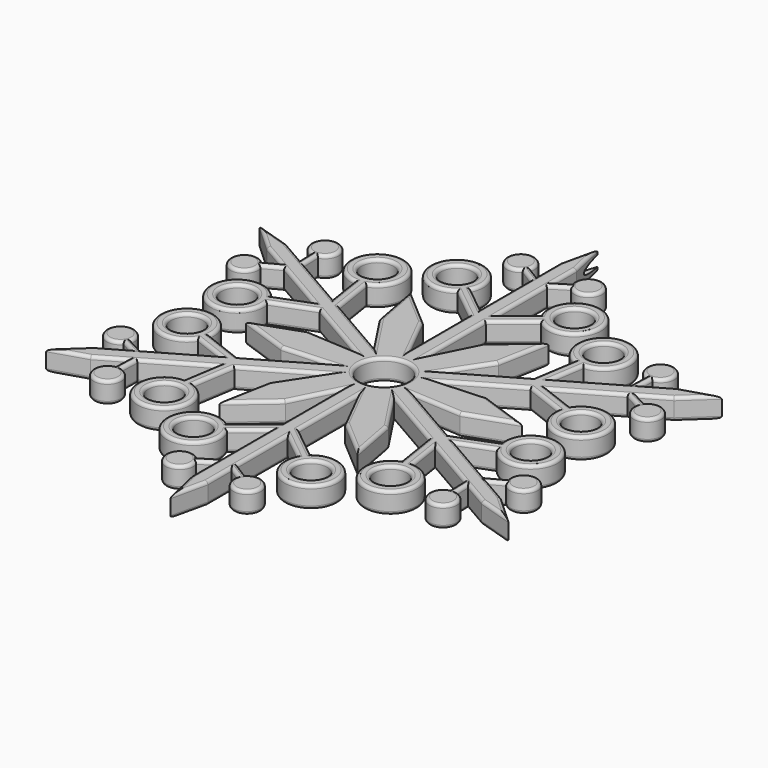
from build123d import *

# Parameters (mm, degrees)
F0_R     = 1.5
F1_DEPTH = 1
F3_COUNT = 6
F4_R     = 2.25
F5_DEPTH = 2.001
F6_R     = 0.29999
F8_R     = 0.5
F9_DEPTH = 3


# Not quite as in the source:
# - a fillet or chamfer is up to 0.001 mm smaller than in the source, because OpenCascade refuses the exact size


with BuildPart() as f1:
    # F0 (on Top) → F1 (new body, symmetric)
    with BuildSketch(Plane.XY):
        with BuildLine():
            Line((0.7675196002, 21.582075705), (0, 25))
            Line((0, 25), (-0.7675196002, 21.582075705))
            Line((-0.7675196002, 21.582075705), (-0.7675196002, 18.8360231686))
            Line((-0.7675196002, 18.8360231686), (-1.9404436058, 19.5647595556))
            ThreePointArc((-1.9404436058, 19.5647595556), (-4.2601998947, 20.6528344986), (-2.2570854353, 19.0551146284))
            Line((-2.2570854353, 19.0551146284), (-0.7675196002, 18.1296490231))
            Line((-0.7675196002, 18.1296490231), (-0.7675196002, 12.2385434307))
            Line((-0.7675196002, 12.2385434307), (-3.2830186101, 14.2674330896))
            ThreePointArc((-3.2830186101, 14.2674330896), (-7.4494710439, 16.9855432476), (-3.9108200753, 13.4890595802))
            Line((-3.9108200753, 13.4890595802), (-0.7675196002, 10.9538131723))
            Line((-0.7675196002, 10.9538131723), (-0.7675196002, 4.0098051105))
            Line((-0.7675196002, 4.0098051105), (-2.8030935325, 8.0551004166))
            Line((-2.8030935325, 8.0551004166), (-6.46553243, 11.1986306667))
            Line((-6.46553243, 11.1986306667), (0, 0))
            Line((0, 0), (6.46553243, 11.1986306667))
            Line((6.46553243, 11.1986306667), (2.8030935325, 8.0551004166))
            Line((2.8030935325, 8.0551004166), (0.7675196002, 4.0098051105))
            Line((0.7675196002, 4.0098051105), (0.7675196002, 10.9538131723))
            Line((0.7675196002, 10.9538131723), (3.9108200753, 13.4890595802))
            ThreePointArc((3.9108200753, 13.4890595802), (7.4494710439, 16.9855432476), (3.2830186101, 14.2674330896))
            Line((3.2830186101, 14.2674330896), (0.7675196002, 12.2385434307))
            Line((0.7675196002, 12.2385434307), (0.7675196002, 18.1296490231))
            Line((0.7675196002, 18.1296490231), (2.2570854353, 19.0551146284))
            ThreePointArc((2.2570854353, 19.0551146284), (4.2601998947, 20.6528344986), (1.9404436058, 19.5647595556))
            Line((1.9404436058, 19.5647595556), (0.7675196002, 18.8360231686))
            Line((0.7675196002, 18.8360231686), (0.7675196002, 21.582075705))
        make_face()
        with Locations((-5.5035372702, 15.4160395845)):
            Circle(F0_R, mode=Mode.SUBTRACT)
        with Locations((5.5035372702, 15.4160395845)):
            Circle(F0_R, mode=Mode.SUBTRACT)
    extrude(amount=F1_DEPTH, both=True)

    # F3: F1 ×6 about axis
    f3_axis = Axis((0, 0, 6.4609721303), (0, 0, 1))


with BuildPart() as f1_1:
    add(f1.part)
    for i in range(1, F3_COUNT):
        add(f1.part.rotate(f3_axis, i * 360 / F3_COUNT))

    # F4 (on face) → F5 (cut, through all)
    with BuildSketch(Plane.XY.offset(1)):
        Circle(F4_R)
    extrude(amount=-F5_DEPTH, mode=Mode.SUBTRACT)

    # F6 (radius 0.3 in the source; OpenCascade refuses exactly that, so slightly less here)
    f6_edges = [f1_1.edges().sort_by_distance(p)[0] for p in [
        (4.2602, 20.652834, 1),
        (1.512303, 18.592382, 1),
        (1.353982, 19.200391, 1),
        (0.76752, 15.184096, 1),
        (0.76752, 20.209049, 1),
        (2.025269, 13.252988, 1),
        (0.38376, 23.291038, 1),
        (7.449471, 16.985543, 1),
        (-0.38376, 23.291038, 1),
        (2.33917, 12.221436, 1),
        (-0.76752, 20.209049, 1),
        (0.76752, 7.481809, 1),
        (-1.353982, 19.200391, 1),
        (1.785307, 6.032453, 1),
        (-4.2602, 20.652834, 1),
        (4.634313, 9.626866, 1),
        (-1.512303, 18.592382, 1),
        (6.019954, 8.826866, 1),
        (-0.76752, 15.184096, 1),
        (4.331604, 4.562347, 1),
        (-2.025269, 13.252988, 1),
        (6.095677, 4.405596, 1),
        (-7.449471, 16.985543, 1),
        (9.414489, 8.136499, 1),
        (-2.33917, 12.221436, 1),
        (10.985176, 14.944203, 1),
        (-0.76752, 7.481809, 1),
        (10.46479, 8.380429, 1),
        (-1.785307, 6.032453, 1),
        (12.766053, 8.25674, 1),
        (-4.634313, 9.626866, 1),
        (15.345324, 10.605883, 1),
        (-6.019954, 8.826866, 1),
        (15.755779, 14.015859, 1),
        (-4.331604, 4.562347, 1),
        (15.951036, 10.772778, 1),
        (-6.095677, 4.405596, 1),
        (17.11779, 10.769216, 1),
        (-9.414489, 8.136499, 1),
        (19.978751, 11.977865, 1),
        (-10.985176, 14.944203, 1),
        (20.36251, 11.313173, 1),
        (-10.46479, 8.380429, 1),
        (17.88531, 9.439833, 1),
        (-12.766053, 8.25674, 1),
        (17.305017, 8.427613, 1),
        (-15.345324, 10.605883, 1),
        (20.015979, 6.636976, 1),
        (-15.755779, 14.015859, 1),
        (16.857626, 7.986499, 1),
        (-15.951036, 10.772778, 1),
        (13.533573, 6.927357, 1),
        (-17.11779, 10.769216, 1),
        (12.490059, 4.87256, 1),
        (-19.978751, 11.977865, 1),
        (18.434647, 2.04134, 1),
        (-20.36251, 11.313173, 1),
        (11.753659, 4.084938, 1),
        (-17.88531, 9.439833, 1),
        (6.863197, 3.076213, 1),
        (-17.305017, 8.427613, 1),
        (6.116911, 1.470106, 1),
        (-20.015979, 6.636976, 1),
        (10.654267, 0.8, 1),
        (-16.857626, 7.986499, 1),
        (10.654267, -0.8, 1),
        (-13.533573, 6.927357, 1),
        (6.116911, -1.470106, 1),
        (-12.490059, 4.87256, 1),
        (6.863197, -3.076213, 1),
        (-18.434647, 2.04134, 1),
        (11.753659, -4.084938, 1),
        (-11.753659, 4.084938, 1),
        (18.434647, -2.04134, 1),
        (-6.863197, 3.076213, 1),
        (12.490059, -4.87256, 1),
        (-6.116911, 1.470106, 1),
        (13.533573, -6.927357, 1),
        (-10.654267, 0.8, 1),
        (16.857626, -7.986499, 1),
        (-10.654267, -0.8, 1),
        (20.015979, -6.636976, 1),
        (-6.116911, -1.470106, 1),
        (17.305017, -8.427613, 1),
        (-6.863197, -3.076213, 1),
        (17.88531, -9.439833, 1),
        (-11.753659, -4.084938, 1),
        (20.36251, -11.313173, 1),
        (-18.434647, -2.04134, 1),
        (19.978751, -11.977865, 1),
        (-12.490059, -4.87256, 1),
        (17.11779, -10.769216, 1),
        (-13.533573, -6.927357, 1),
        (15.951036, -10.772778, 1),
        (-16.857626, -7.986499, 1),
        (15.755779, -14.015859, 1),
        (-20.015979, -6.636976, 1),
        (15.345324, -10.605883, 1),
        (-17.305017, -8.427613, 1),
        (12.766053, -8.25674, 1),
        (-17.88531, -9.439833, 1),
        (10.46479, -8.380429, 1),
        (-20.36251, -11.313173, 1),
        (10.985176, -14.944203, 1),
        (-19.978751, -11.977865, 1),
        (9.414489, -8.136499, 1),
        (-17.11779, -10.769216, 1),
        (6.095677, -4.405596, 1),
        (-15.951036, -10.772778, 1),
        (4.331604, -4.562347, 1),
        (-15.755779, -14.015859, 1),
        (6.019954, -8.826866, 1),
        (-15.345324, -10.605883, 1),
        (4.634313, -9.626866, 1),
        (-12.766053, -8.25674, 1),
        (1.785307, -6.032453, 1),
        (-10.46479, -8.380429, 1),
        (0.76752, -7.481809, 1),
        (-10.985176, -14.944203, 1),
        (2.33917, -12.221436, 1),
        (-9.414489, -8.136499, 1),
        (7.449471, -16.985543, 1),
        (-6.095677, -4.405596, 1),
        (2.025269, -13.252988, 1),
        (-4.331604, -4.562347, 1),
        (0.76752, -15.184096, 1),
        (-6.019954, -8.826866, 1),
        (1.512303, -18.592382, 1),
        (-4.634313, -9.626866, 1),
        (4.2602, -20.652834, 1),
        (-1.785307, -6.032453, 1),
        (1.353982, -19.200391, 1),
        (-0.76752, -7.481809, 1),
        (0.76752, -20.209049, 1),
        (-2.33917, -12.221436, 1),
        (0.38376, -23.291038, 1),
        (-7.449471, -16.985543, 1),
        (-0.38376, -23.291038, 1),
        (-2.025269, -13.252988, 1),
        (-0.76752, -20.209049, 1),
        (-0.76752, -15.184096, 1),
        (-1.353982, -19.200391, 1),
        (-1.512303, -18.592382, 1),
        (-4.2602, -20.652834, 1),
        (-9.848913, -13.773261, 1),
        (-4.003537, -15.41604, 1),
        (-15.352451, -4.240855, 1),
        (7.003537, -15.41604, 1),
        (11.348913, -11.175185, 1),
        (16.852451, -1.642779, 1),
        (-16.852451, 1.642779, 1),
        (-11.348913, 11.175185, 1),
        (-7.003537, 15.41604, 1),
        (-2.25, 0, 1),
        (15.352451, 4.240855, 1),
        (4.003537, 15.41604, 1),
        (9.848913, 13.773261, 1),
        (4.2602, 20.652834, -1),
        (1.512303, 18.592382, -1),
        (1.353982, 19.200391, -1),
        (0.76752, 15.184096, -1),
        (0.76752, 20.209049, -1),
        (2.025269, 13.252988, -1),
        (0.38376, 23.291038, -1),
        (7.449471, 16.985543, -1),
        (-0.38376, 23.291038, -1),
        (2.33917, 12.221436, -1),
        (-0.76752, 20.209049, -1),
        (0.76752, 7.481809, -1),
        (-1.353982, 19.200391, -1),
        (1.785307, 6.032453, -1),
        (-4.2602, 20.652834, -1),
        (4.634313, 9.626866, -1),
        (-1.512303, 18.592382, -1),
        (6.019954, 8.826866, -1),
        (-0.76752, 15.184096, -1),
        (4.331604, 4.562347, -1),
        (-2.025269, 13.252988, -1),
        (6.095677, 4.405596, -1),
        (-7.449471, 16.985543, -1),
        (9.414489, 8.136499, -1),
        (-2.33917, 12.221436, -1),
        (10.985176, 14.944203, -1),
        (-0.76752, 7.481809, -1),
        (10.46479, 8.380429, -1),
        (-1.785307, 6.032453, -1),
        (12.766053, 8.25674, -1),
        (-4.634313, 9.626866, -1),
        (15.345324, 10.605883, -1),
        (-6.019954, 8.826866, -1),
        (15.755779, 14.015859, -1),
        (-4.331604, 4.562347, -1),
        (15.951036, 10.772778, -1),
        (-6.095677, 4.405596, -1),
        (17.11779, 10.769216, -1),
        (-9.414489, 8.136499, -1),
        (19.978751, 11.977865, -1),
        (-10.985176, 14.944203, -1),
        (20.36251, 11.313173, -1),
        (-10.46479, 8.380429, -1),
        (17.88531, 9.439833, -1),
        (-12.766053, 8.25674, -1),
        (17.305017, 8.427613, -1),
        (-15.345324, 10.605883, -1),
        (20.015979, 6.636976, -1),
        (-15.755779, 14.015859, -1),
        (16.857626, 7.986499, -1),
        (-15.951036, 10.772778, -1),
        (13.533573, 6.927357, -1),
        (-17.11779, 10.769216, -1),
        (12.490059, 4.87256, -1),
        (-19.978751, 11.977865, -1),
        (18.434647, 2.04134, -1),
        (-20.36251, 11.313173, -1),
        (11.753659, 4.084938, -1),
        (-17.88531, 9.439833, -1),
        (6.863197, 3.076213, -1),
        (-17.305017, 8.427613, -1),
        (6.116911, 1.470106, -1),
        (-20.015979, 6.636976, -1),
        (10.654267, 0.8, -1),
        (-16.857626, 7.986499, -1),
        (10.654267, -0.8, -1),
        (-13.533573, 6.927357, -1),
        (6.116911, -1.470106, -1),
        (-12.490059, 4.87256, -1),
        (6.863197, -3.076213, -1),
        (-18.434647, 2.04134, -1),
        (11.753659, -4.084938, -1),
        (-11.753659, 4.084938, -1),
        (18.434647, -2.04134, -1),
        (-6.863197, 3.076213, -1),
        (12.490059, -4.87256, -1),
        (-6.116911, 1.470106, -1),
        (13.533573, -6.927357, -1),
        (-10.654267, 0.8, -1),
        (16.857626, -7.986499, -1),
        (-10.654267, -0.8, -1),
        (20.015979, -6.636976, -1),
        (-6.116911, -1.470106, -1),
        (17.305017, -8.427613, -1),
        (-6.863197, -3.076213, -1),
        (17.88531, -9.439833, -1),
        (-11.753659, -4.084938, -1),
        (20.36251, -11.313173, -1),
        (-18.434647, -2.04134, -1),
        (19.978751, -11.977865, -1),
        (-12.490059, -4.87256, -1),
        (17.11779, -10.769216, -1),
        (-13.533573, -6.927357, -1),
        (15.951036, -10.772778, -1),
        (-16.857626, -7.986499, -1),
        (15.755779, -14.015859, -1),
        (-20.015979, -6.636976, -1),
        (15.345324, -10.605883, -1),
        (-17.305017, -8.427613, -1),
        (12.766053, -8.25674, -1),
        (-17.88531, -9.439833, -1),
        (10.46479, -8.380429, -1),
        (-20.36251, -11.313173, -1),
        (10.985176, -14.944203, -1),
        (-19.978751, -11.977865, -1),
        (9.414489, -8.136499, -1),
        (-17.11779, -10.769216, -1),
        (6.095677, -4.405596, -1),
        (-15.951036, -10.772778, -1),
        (4.331604, -4.562347, -1),
        (-15.755779, -14.015859, -1),
        (6.019954, -8.826866, -1),
        (-15.345324, -10.605883, -1),
        (4.634313, -9.626866, -1),
        (-12.766053, -8.25674, -1),
        (1.785307, -6.032453, -1),
        (-10.46479, -8.380429, -1),
        (0.76752, -7.481809, -1),
        (-10.985176, -14.944203, -1),
        (2.33917, -12.221436, -1),
        (-9.414489, -8.136499, -1),
        (7.449471, -16.985543, -1),
        (-6.095677, -4.405596, -1),
        (2.025269, -13.252988, -1),
        (-4.331604, -4.562347, -1),
        (0.76752, -15.184096, -1),
        (-6.019954, -8.826866, -1),
        (1.512303, -18.592382, -1),
        (-4.634313, -9.626866, -1),
        (4.2602, -20.652834, -1),
        (-1.785307, -6.032453, -1),
        (1.353982, -19.200391, -1),
        (-0.76752, -7.481809, -1),
        (0.76752, -20.209049, -1),
        (-2.33917, -12.221436, -1),
        (0.38376, -23.291038, -1),
        (-7.449471, -16.985543, -1),
        (-0.38376, -23.291038, -1),
        (-2.025269, -13.252988, -1),
        (-0.76752, -20.209049, -1),
        (-0.76752, -15.184096, -1),
        (-1.353982, -19.200391, -1),
        (-1.512303, -18.592382, -1),
        (-4.2602, -20.652834, -1),
        (-9.848913, -13.773261, -1),
        (-4.003537, -15.41604, -1),
        (-15.352451, -4.240855, -1),
        (7.003537, -15.41604, -1),
        (11.348913, -11.175185, -1),
        (16.852451, -1.642779, -1),
        (-16.852451, 1.642779, -1),
        (-11.348913, 11.175185, -1),
        (-7.003537, 15.41604, -1),
        (-2.25, 0, -1),
        (15.352451, 4.240855, -1),
        (4.003537, 15.41604, -1),
        (9.848913, 13.773261, -1),
    ]]
    fillet(f6_edges, radius=F6_R)

    # F8 (on offset) → F9 (cut)
    with BuildSketch(Plane.XZ.offset(-25)):
        Circle(F8_R)
    extrude(amount=F9_DEPTH, mode=Mode.SUBTRACT)


solid = f1_1.part
